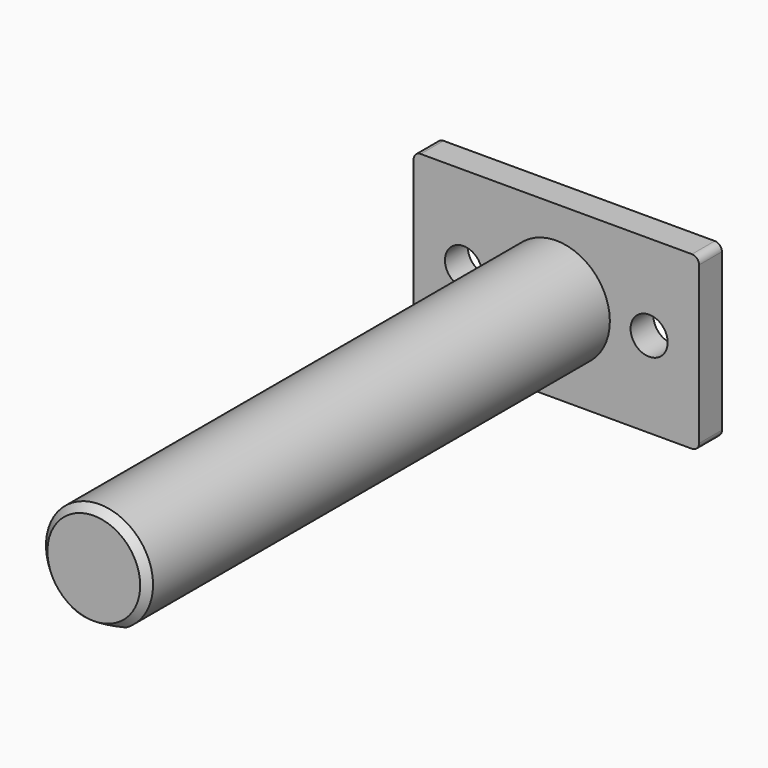
from build123d import *

# Parameters (mm, degrees)
F0_W     = 40
F0_H     = 24
F0_R     = 7.5
F1_DEPTH = 2
F2_DEPTH = 83
F4_D     = 5.2
F4_DEPTH = 15
F4_TIP   = 1.5622376095
F6_DEPTH = 75
F8_DEPTH = 75
F9_SIZE  = 0.99999
F10_R    = 1


# Not quite as in the source:
# - a fillet or chamfer is up to 0.001 mm smaller than in the source, because OpenCascade refuses the exact size


with BuildPart() as f1:
    # F0 (on Front) → F1 (new body, symmetric)
    with BuildSketch(Plane.XZ):
        Rectangle(F0_W, F0_H)
        Circle(F0_R, mode=Mode.SUBTRACT)
    extrude(amount=F1_DEPTH, both=True)

    # F0 (on Front) → F2 (join)
    with BuildSketch(Plane.XZ):
        Circle(F0_R)
    extrude(amount=F2_DEPTH)

    # F4
    with Locations(Plane(origin=(0, 2, 0), x_dir=(-1, 0, 0), z_dir=(0, 1, 0))):
        with Locations((-13, 0), (13, 0)):
            Hole(F4_D / 2, depth=F4_DEPTH)
            with Locations((0, 0, -(F4_DEPTH + F4_TIP / 2))):  # 118° drill point
                Cone(0, F4_D / 2, F4_TIP, mode=Mode.SUBTRACT)

    # F5 (on Front) → F6 (cut)
    with BuildSketch(Plane.XZ):
        with BuildLine():
            Line((3.7416573868, -6.5), (-3.7416573868, -6.5))
            ThreePointArc((-3.7416573868, -6.5), (0, -7.5), (3.7416573868, -6.5))
        make_face()
    extrude(amount=-F6_DEPTH, mode=Mode.SUBTRACT)

    # F7 (on face) → F8 (cut)
    with BuildSketch(Plane.XZ.offset(83)):
        with BuildLine():
            ThreePointArc((-3.7416573868, -6.5), (0, -7.5), (3.7416573868, -6.5))
            Line((3.7416573868, -6.5), (-3.7416573868, -6.5))
        make_face()
    extrude(amount=-F8_DEPTH, mode=Mode.SUBTRACT)

    # F9 (size 1 in the source; OpenCascade refuses exactly that, so slightly less here)
    f9_edges = [f1.edges().sort_by_distance(p)[0] for p in [
        (-7.5, 2, 0),
        (-3.754169, -83, 6.492782),
    ]]
    chamfer(f9_edges, length=F9_SIZE)

    # F10
    f10_edges = [f1.edges().sort_by_distance(p)[0] for p in [
        (20, 0, 12),
        (-20, 0, 12),
        (20, 0, -12),
        (-20, 0, -12),
    ]]
    fillet(f10_edges, radius=F10_R)


solid = f1.part
